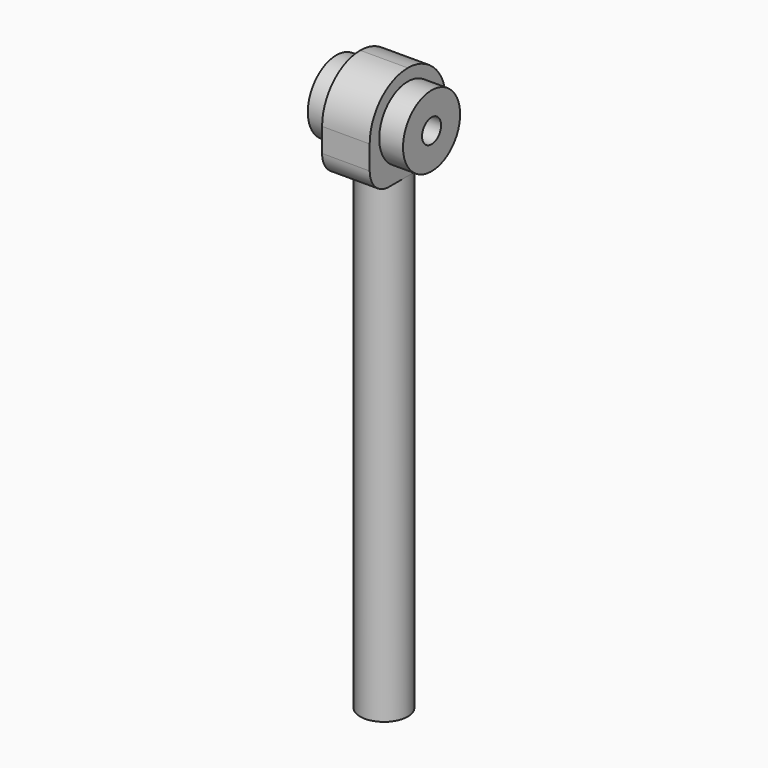
from build123d import *

# Parameters (mm, degrees)
F0_R          = 6.35
F1_DEPTH      = 127
F2_W          = 12.7
F2_H          = 25.4
F3_DEPTH      = 25.4
F4_R          = 9.525
F4_R_2        = 3.175
F5_DEPTH      = 6.35
F5_DEPTH_BACK = 19.05
F6_DEPTH      = 25.4
F7_R          = 6.34999
F8_R          = 12.69999


# Not quite as in the source:
# - a fillet or chamfer is up to 0.001 mm smaller than in the source, because OpenCascade refuses the exact size


with BuildPart() as f1:
    # F0 (on Top) → F1 (new body)
    with BuildSketch(Plane.XY):
        Circle(F0_R)
    extrude(amount=F1_DEPTH)

    # F2 (on face) → F3 (join)
    with BuildSketch(Plane.XY.offset(127)):
        Rectangle(F2_W, F2_H)
    extrude(amount=F3_DEPTH)

    # F4 (on face) → F5 (join, two sides)
    with BuildSketch(Plane.YZ.offset(6.35)) as f5_sk:
        with Locations((0, 139.7)):
            Circle(F4_R)
        with Locations((0, 139.7)):
            Circle(F4_R_2, mode=Mode.SUBTRACT)
    extrude(amount=F5_DEPTH)
    extrude(f5_sk.sketch, amount=-F5_DEPTH_BACK)

    # F6 (cut): a face of the model
    f6_faces = [f1.faces().sort_by_distance(p)[0] for p in [
        (6.35, 0, 139.7),
    ]]
    extrude(f6_faces, amount=-F6_DEPTH, mode=Mode.SUBTRACT)

    # F7 (radius 6.35 in the source; OpenCascade refuses exactly that, so slightly less here)
    f7_edges = [f1.edges().sort_by_distance(p)[0] for p in [
        (0, -12.7, 127),
        (0, 12.7, 127),
    ]]
    fillet(f7_edges, radius=F7_R)

    # F8 (radius 12.7 in the source; OpenCascade refuses exactly that, so slightly less here)
    f8_edges = [f1.edges().sort_by_distance(p)[0] for p in [
        (0, -12.7, 152.4),
        (0, 12.7, 152.4),
    ]]
    fillet(f8_edges, radius=F8_R)


solid = f1.part
